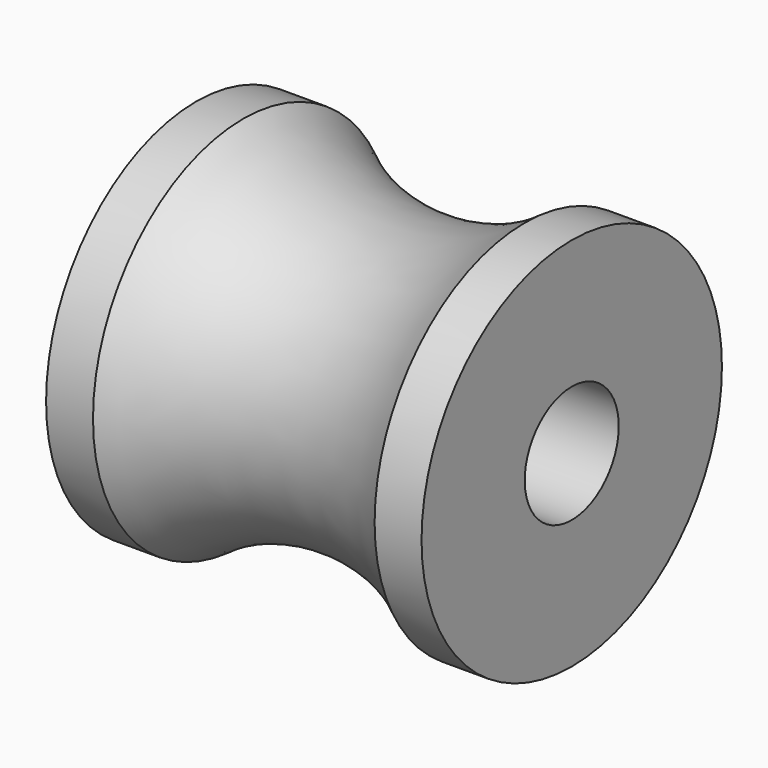
from build123d import *


# Not quite as in the source:
# - a feature names something its author has since deleted; it is built from what else it names


with BuildPart() as f1:
    # F0 (on Front) → F1 (revolve)
    with BuildSketch(Plane.XZ):
        with BuildLine():
            Line((-12.7, 12.7), (-12.7, 3.9751))
            Line((-12.7, 3.9751), (12.7, 3.9751))
            Line((12.7, 3.9751), (12.7, 12.7))
            Line((12.7, 12.7), (9.525, 12.7))
            ThreePointArc((9.525, 12.7), (0, 9.525), (-9.525, 12.7))
            Line((-9.525, 12.7), (-12.7, 12.7))
        make_face()
    revolve(axis=Axis((2.2681517906, 0, 0), (1, 0, 0)))


solid = f1.part
